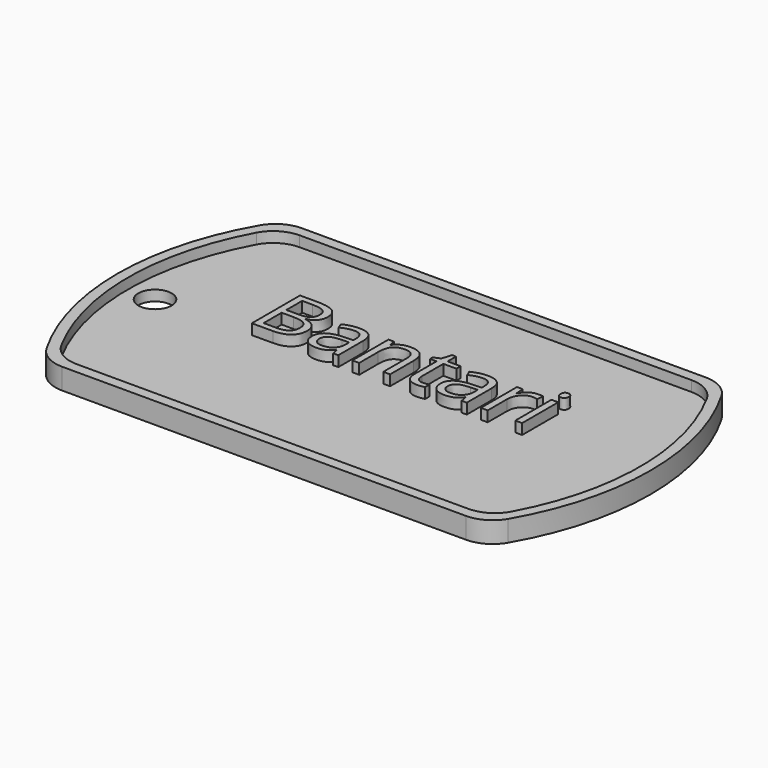
from build123d import *

# Parameters (mm, degrees)
F1_DEPTH     = 1
F3_DEPTH     = 1
F4_R         = 1.5875
F5_DEPTH     = 1
F6_TEXT_SIZE = 8.0385390902
F7_DEPTH     = 1


# Not quite as in the source:
# - Text() gives the source's letters only with a copy of the font that has no kerning and outlines rounded to 1/6400 em; it was checked with that copy


with BuildPart() as f1:
    # F0 (on Top) → F1 (new body)
    with BuildSketch(Plane.XY):
        with BuildLine():
            ThreePointArc((-19.2474145991, 14.2875), (-20.8349145991, 13.862130657), (-21.9970452561, 12.7))
            ThreePointArc((-21.9970452561, 12.7), (-25.4, 0), (-21.9970452561, -12.7))
            ThreePointArc((-21.9970452561, -12.7), (-20.8349145991, -13.862130657), (-19.2474145991, -14.2875))
            Line((-19.2474145991, -14.2875), (19.2474145991, -14.2875))
            ThreePointArc((19.2474145991, -14.2875), (20.8349145991, -13.862130657), (21.9970452561, -12.7))
            ThreePointArc((21.9970452561, -12.7), (25.4, 0), (21.9970452561, 12.7))
            ThreePointArc((21.9970452561, 12.7), (20.8349145991, 13.862130657), (19.2474145991, 14.2875))
            Line((19.2474145991, 14.2875), (-19.2474145991, 14.2875))
        make_face()
    extrude(amount=F1_DEPTH)

    # F2 (on face) → F3 (join)
    with BuildSketch(Plane.XY.offset(1)):
        with BuildLine():
            Line((19.2474145991, 14.2875), (-19.2474145991, 14.2875))
            ThreePointArc((-19.2474145991, 14.2875), (-20.8349145991, 13.862130657), (-21.9970452561, 12.7))
            ThreePointArc((-21.9970452561, 12.7), (-25.4, 0), (-21.9970452561, -12.7))
            ThreePointArc((-21.9970452561, -12.7), (-20.8349145991, -13.862130657), (-19.2474145991, -14.2875))
            Line((-19.2474145991, -14.2875), (19.2474145991, -14.2875))
            ThreePointArc((19.2474145991, -14.2875), (20.8349145991, -13.862130657), (21.9970452561, -12.7))
            ThreePointArc((21.9970452561, -12.7), (25.4, 0), (21.9970452561, 12.7))
            ThreePointArc((21.9970452561, 12.7), (20.8349145991, 13.862130657), (19.2474145991, 14.2875))
        make_face()
        with BuildLine():
            ThreePointArc((-21.4526124879, 11.6252061249), (-20.2856017842, 12.8404540819), (-18.6611352482, 13.2875))
            Line((-18.6611352482, 13.2875), (18.6611352482, 13.2875))
            ThreePointArc((18.6611352482, 13.2875), (20.2856017842, 12.8404540819), (21.4526124879, 11.6252061249))
            ThreePointArc((21.4526124879, 11.6252061249), (24.4, 0), (21.4526124879, -11.6252061249))
            ThreePointArc((21.4526124879, -11.6252061249), (20.2856017842, -12.8404540819), (18.6611352482, -13.2875))
            Line((18.6611352482, -13.2875), (-18.6611352482, -13.2875))
            ThreePointArc((-18.6611352482, -13.2875), (-20.2856017842, -12.8404540819), (-21.4526124879, -11.6252061249))
            ThreePointArc((-21.4526124879, -11.6252061249), (-24.4, 0), (-21.4526124879, 11.6252061249))
        make_face(mode=Mode.SUBTRACT)
    extrude(amount=F3_DEPTH)

    # F4 (on face) → F5 (cut)
    with BuildSketch(Plane.XY.offset(1)):
        with Locations((-21.821282804, 0)):
            Circle(F4_R)
    extrude(amount=-F5_DEPTH, mode=Mode.SUBTRACT)

    # F6 (on face) → F7 (join)
    with BuildSketch(Plane.XY.offset(1)):
        with Locations((-13.3820818737, 0)):
            Text('Bantari', F6_TEXT_SIZE, font='Open Sans', text_align=(TextAlign.LEFT, TextAlign.BOTTOM))
    extrude(amount=F7_DEPTH)


solid = f1.part
